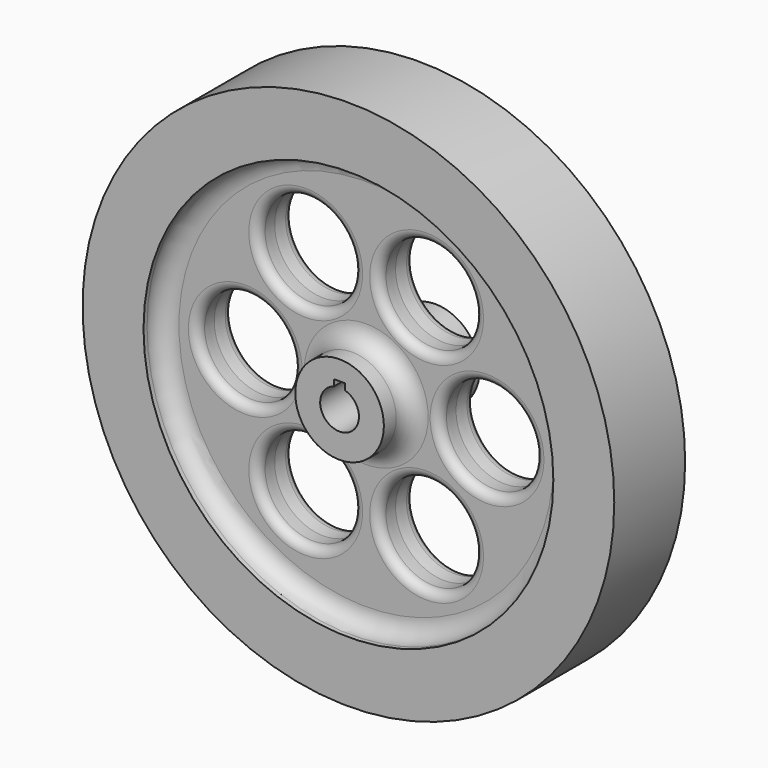
from build123d import *

# Parameters (mm, degrees)
F0_R          = 76.2
F0_R_2        = 58.7375
F1_DEPTH      = 12.7
F1_DEPTH_BACK = 12.7
F0_R_3        = 12.7
F2_DEPTH      = 15.875
F2_DEPTH_BACK = 18.415
F3_R          = 62.6663384898
F3_R_2        = 13.97
F3_R_3        = 9.4882721097
F4_DEPTH      = 6.35
F4_TAPER      = -3
F4_DEPTH_BACK = 6.35
F4_TAPER_BACK = -3
F6_R          = 5.08
F7_R          = 2.54


with BuildPart() as f1:
    # F0 (on Front) → F1 (new body, two sides)
    with BuildSketch(Plane.XZ) as f1_sk:
        Circle(F0_R)
        Circle(F0_R_2, mode=Mode.SUBTRACT)
    extrude(amount=F1_DEPTH)
    extrude(f1_sk.sketch, amount=-F1_DEPTH_BACK)



with BuildPart() as f2:
    # F0 (on Front) → F2 (new body, two sides)
    with BuildSketch(Plane.XZ) as f2_sk:
        Circle(F0_R_3)
        with BuildLine():
            ThreePointArc((1.5875, 5.3246368714), (0, -5.55625), (-1.5875, 5.3246368714))
            Line((-1.5875, 5.3246368714), (-1.5875, 7.14375))
            Line((-1.5875, 7.14375), (1.5875, 7.14375))
            Line((1.5875, 7.14375), (1.5875, 5.3246368714))
        make_face(mode=Mode.SUBTRACT)
    extrude(amount=F2_DEPTH)
    extrude(f2_sk.sketch, amount=-F2_DEPTH_BACK)


with BuildPart() as f1_1:
    add(f1.part)

    add(f2.part)  # F4 merges F2
    # F3 (on face) → F4 (join, two sides)
    with BuildSketch(Plane.XZ) as f4_sk:
        Circle(F3_R)
        with Locations((-17.3283684999, -30.0136146541)):
            Circle(F3_R_2, mode=Mode.SUBTRACT)
        with Locations((17.3283684999, -30.0136146541)):
            Circle(F3_R_2, mode=Mode.SUBTRACT)
        with Locations((-34.6567369998, 0)):
            Circle(F3_R_2, mode=Mode.SUBTRACT)
        with Locations((-17.3283684999, 30.0136146541)):
            Circle(F3_R_2, mode=Mode.SUBTRACT)
        Circle(F3_R_3, mode=Mode.SUBTRACT)
        with Locations((17.3283684999, 30.0136146541)):
            Circle(F3_R_2, mode=Mode.SUBTRACT)
        with Locations((34.6567369998, 0)):
            Circle(F3_R_2, mode=Mode.SUBTRACT)
    extrude(amount=F4_DEPTH, taper=F4_TAPER)
    extrude(f4_sk.sketch, amount=-F4_DEPTH_BACK, taper=F4_TAPER_BACK)

    # F5: union 

    # F6
    f6_edges = [f1_1.edges().sort_by_distance(p)[0] for p in [
        (-58.7375, 6.35, 0),
        (-12.7, 6.35, 0),
        (-12.7, -6.35, 0),
        (-58.7375, -6.35, 0),
    ]]
    fillet(f6_edges, radius=F6_R)

    # F7
    f7_edges = [f1_1.edges().sort_by_distance(p)[0] for p in [
        (-30.965579, -6.35, -30.013615),
        (3.691158, -6.35, -30.013615),
        (-48.293948, -6.35, 0),
        (-30.965579, -6.35, 30.013615),
        (21.019526, -6.35, 0),
        (3.691158, -6.35, 30.013615),
        (-30.965579, 6.35, -30.013615),
        (3.691158, 6.35, -30.013615),
        (-48.293948, 6.35, 0),
        (-30.965579, 6.35, 30.013615),
        (21.019526, 6.35, 0),
        (3.691158, 6.35, 30.013615),
    ]]
    fillet(f7_edges, radius=F7_R)


solid = f1_1.part
